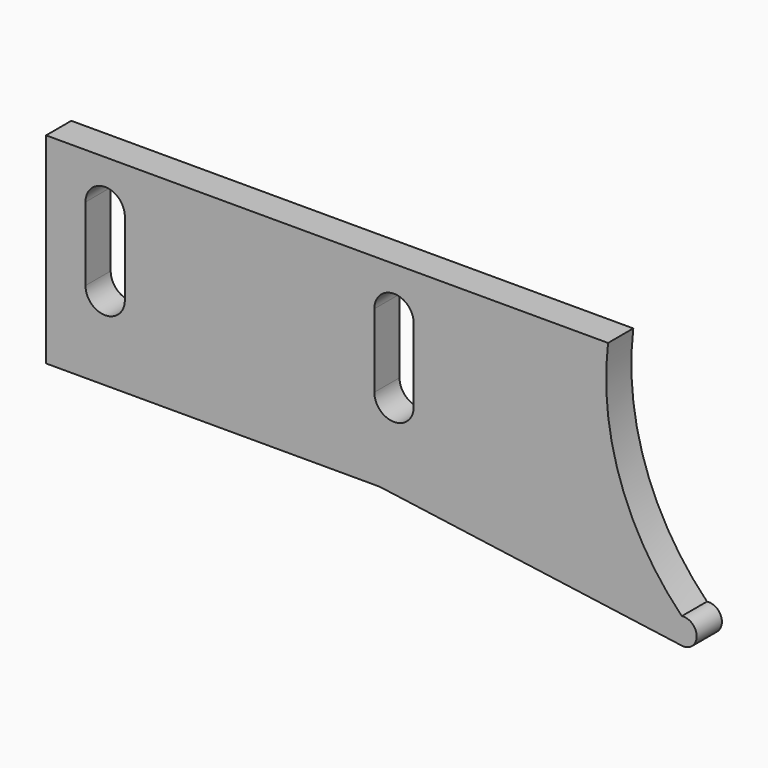
from build123d import *

# Parameters (mm, degrees)
F1_DEPTH = 12


# Not quite as in the source:
# - a feature names something its author has since deleted; it is built from what else it names


with BuildPart() as f1:
    # F0 (on Front) → F1 (new body)
    with BuildSketch(Plane.XZ):
        with BuildLine():
            Line((-78.3512531443, 52.5226152241), (-78.3512531443, -23.4773847759))
            Line((-78.3512531443, -23.4773847759), (48.6487468557, -23.4773847759))
            Line((48.6487468557, -23.4773847759), (163.7198627451, -39.3522962011))
            ThreePointArc((163.7198627451, -39.3522962011), (169.4031778605, -34.3992082296), (163.7198627451, -29.4461202581))
            ThreePointArc((163.7198627451, -29.4461202581), (140.2372169997, 8.5604113595), (135.6487468557, 53))
            Line((135.6487468557, 53), (129.9201593475, 53))
            Line((129.9201593475, 53), (-55.8512531443, 53))
            Line((-55.8512531443, 53), (-78.3512531443, 53))
            Line((-78.3512531443, 53), (-78.3512531443, 52.5226152241))
        make_face()
        with BuildLine():
            Line((-63.3512531443, 7.5), (-63.3512531443, 21.5))
            Line((-63.3512531443, 21.5), (-63.3512531443, 35.5))
            ThreePointArc((-63.3512531443, 35.5), (-55.8512531443, 43), (-48.3512531443, 35.5))
            Line((-48.3512531443, 35.5), (-48.3512531443, 7.5))
            ThreePointArc((-48.3512531443, 7.5), (-55.8512531443, 0), (-63.3512531443, 7.5))
        make_face(mode=Mode.SUBTRACT)
        with BuildLine():
            Line((46.6487468557, 7.5), (46.6487468557, 21.5))
            Line((46.6487468557, 21.5), (46.6487468557, 35.5))
            ThreePointArc((46.6487468557, 35.5), (54.1487468557, 43), (61.6487468557, 35.5))
            Line((61.6487468557, 35.5), (61.6487468557, 7.5))
            ThreePointArc((61.6487468557, 7.5), (54.1487468557, 0), (46.6487468557, 7.5))
        make_face(mode=Mode.SUBTRACT)
    extrude(amount=F1_DEPTH)


solid = f1.part
